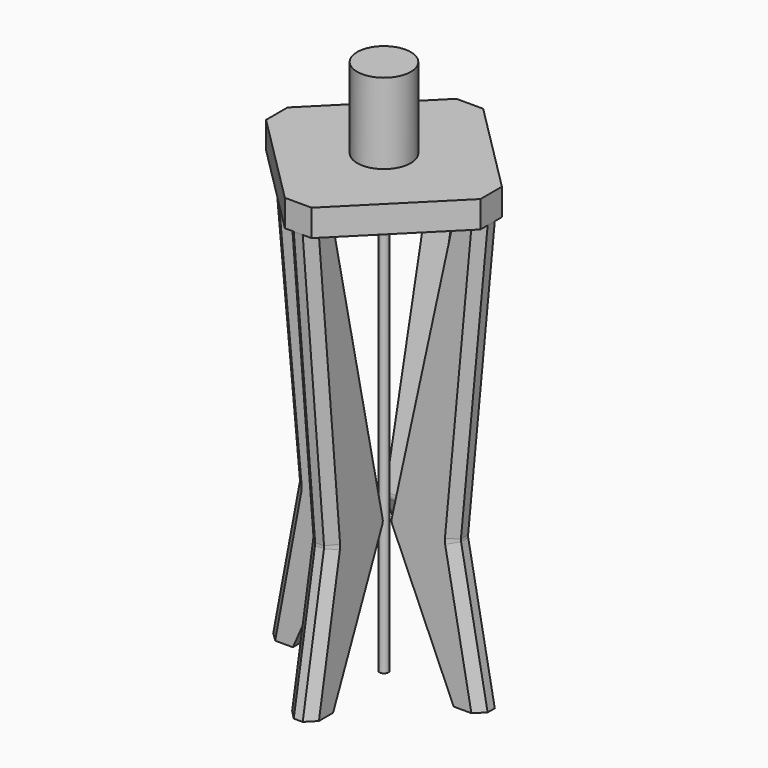
from build123d import *

# Parameters (mm, degrees)
F2_DEPTH  = 9.525
F3_R      = 6.35
F4_R      = 3.175
F5_DEPTH  = 304.8
F8_SIZE   = 6.35
F10_COUNT = 4
F12_DEPTH = 19.05


# Not quite as in the source:
# - a feature of the source that left no trace in its solid (it failed there, or was rolled back) is left out
# - the program builds the solid bodies; features that only make, move or delete a surface that nothing else refers to are left out


with BuildPart() as f2:
    # F1 (on Front) → F2 (new body, symmetric)
    with BuildSketch(Plane.XZ):
        Polygon((-57.15, 101.6), (-76.2, 0), (-57.15, 0), (-12.7, 101.6), (-57.15, 304.8), (-76.2, 304.8), align=None)
    extrude(amount=F2_DEPTH, both=True)

    # F3
    f3_edges = [f2.edges().sort_by_distance(p)[0] for p in [
        (-57.15, 0, 101.6),
        (-12.7, 0, 101.6),
    ]]
    fillet(f3_edges, radius=F3_R)

    # F8
    f8_edges = [f2.edges().sort_by_distance(p)[0] for p in [
        (-66.716586, -9.525, 203.643579),
        (-66.716586, 9.525, 203.643579),
        (-66.757105, 9.525, 50.362106),
        (-66.757105, -9.525, 50.362106),
        (-57.212147, 9.525, 101.602857),
        (-57.212147, -9.525, 101.602857),
    ]]
    chamfer(f8_edges, length=F8_SIZE)


with BuildPart() as f5:
    # F4 (on Top) → F5 (new body, through all)
    with BuildSketch(Plane.XY):
        Circle(F4_R)
    extrude(amount=F5_DEPTH)

    # F0 (on Front) → F6 (revolve)
    with BuildSketch(Plane.XZ):
        Polygon((-19.05, 323.85), (-9.525, 323.85), (0, 323.85), (0, 381), (-19.05, 381), align=None)
        Polygon((-9.525, 323.85), (-9.525, 304.8), (-4.7625, 304.8), (0, 304.8), (0, 323.85), align=None)
    revolve(axis=Axis((0, 0, 352.425), (0, 0, -1)))


with BuildPart() as f10_1:
    # F10: instance of F2
    add(f2.part.rotate(Axis((0, 0, 152.4), (0, 0, -1)), 1 * 360 / F10_COUNT))


with BuildPart() as f10_2:
    # F10: instance of F2
    add(f2.part.rotate(Axis((0, 0, 152.4), (0, 0, -1)), 2 * 360 / F10_COUNT))


with BuildPart() as f10_3:
    # F10: instance of F2
    add(f2.part.rotate(Axis((0, 0, 152.4), (0, 0, -1)), 3 * 360 / F10_COUNT))


with BuildPart() as f12:
    # F11 (on face) → F12 (new body)
    with BuildSketch(Plane.XY.offset(304.8)):
        Polygon((9.525, 76.2), (-9.525, 76.2), (-76.2, 9.525), (-76.2, -9.525), (-9.525, -76.2), (9.525, -76.2), (76.2, -9.525), (76.2, 9.525), align=None)
    extrude(amount=F12_DEPTH)


solid = Compound([f2.part, f5.part, f10_1.part, f10_2.part, f10_3.part, f12.part])
